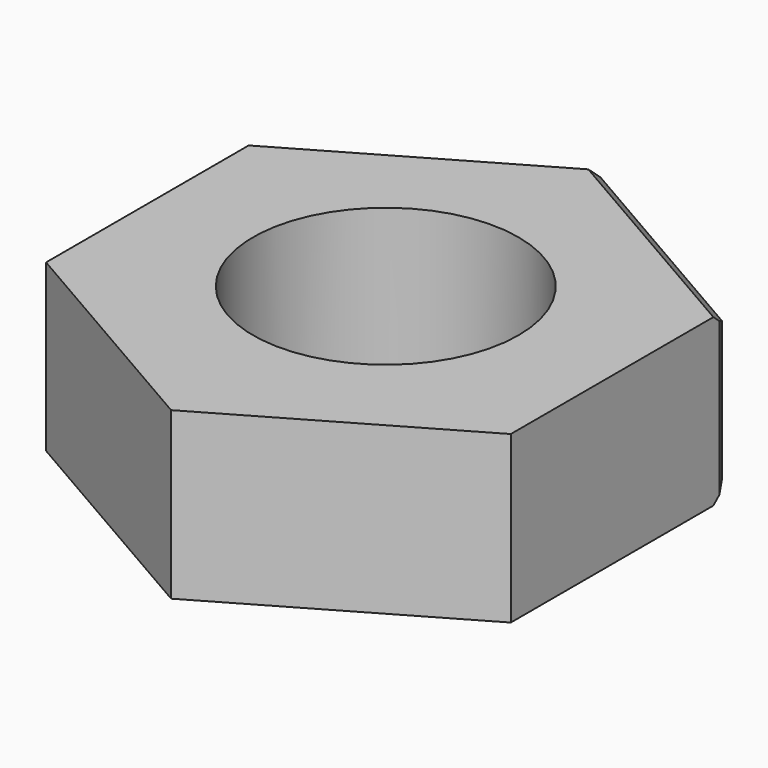
from build123d import *

# Parameters (mm, degrees)
F0_R        = 50.8
F1_DEPTH    = 63.5
F2_T1_DEPTH = 128.3697077416
F2_T3_DEPTH = 128.3697077416
F2_T5_DEPTH = 78.8079500043


# Not quite as in the source:
# - a fillet or chamfer that OpenCascade refuses, or shapes differently, is made with other operations: its cross-section is extruded or revolved along the edge and cut away or added


with BuildPart() as f1:
    # F0 (on Top) → F1 (new body)
    with BuildSketch(Plane.XY):
        Polygon((-88.9, -51.326438931), (0, -102.6528778619), (88.9, -51.326438931), (88.9, 51.326438931), (0, 102.6528778619), (-88.9, 51.326438931), align=None)
        Circle(F0_R, mode=Mode.SUBTRACT)
    extrude(amount=F1_DEPTH)

    # F2: chamfer of 5 on 6 edges, made by hand

    # F2_s2 → F2_t1 (cut)
    with BuildSketch(Plane(origin=(55.5857139903, -32.0924269354, 0), x_dir=(0, 0, 1), z_dir=(-0.8660254038, 0.5, 0))):
        Polygon((58.5, 88.9), (63.5, 83.9), (63.5, 88.9), align=None)
        Polygon((5, 88.9), (0, 83.9), (0, 88.9), align=None)
    extrude(amount=F2_T1_DEPTH, mode=Mode.SUBTRACT)

    # F2_s4 → F2_t3 (cut)
    with BuildSketch(Plane(origin=(55.5857139903, 32.0924269354, 0), x_dir=(0, 0, 1), z_dir=(-0.8660254038, -0.5, 0))):
        Polygon((58.5, 88.9), (63.5, 83.9), (63.5, 88.9), align=None)
        Polygon((5, 88.9), (0, 83.9), (0, 88.9), align=None)
    extrude(amount=F2_T3_DEPTH, mode=Mode.SUBTRACT)

    # F2_s6 → F2_t5 (cut)
    with BuildSketch(Plane.XY.offset(-7.6539750021)):
        Polygon((-88.9, 48.439687585), (-86.4, 52.7698146039), (-88.9, 51.326438931), align=None)
        Polygon((88.9, 48.439687585), (86.4, 52.7698146039), (88.9, 51.326438931), align=None)
    extrude(amount=F2_T5_DEPTH, mode=Mode.SUBTRACT)


solid = f1.part
